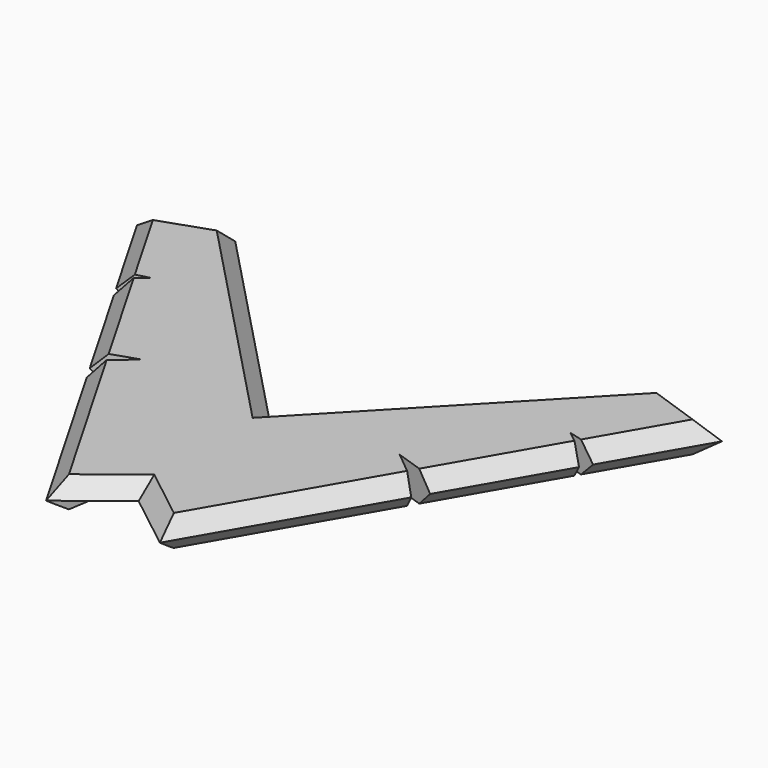
from build123d import *

# Parameters (mm, degrees)
F1_DEPTH = 6.35
F3_DEPTH = 3.175
F4_SIZE  = 3.17499


# Not quite as in the source:
# - a fillet or chamfer is up to 0.001 mm smaller than in the source, because OpenCascade refuses the exact size


with BuildPart() as f1:
    # F0 (on Top) → F1 (new body)
    with BuildSketch(Plane.XY):
        Polygon((-21.1028610796, 36.5512275749), (-11.7370359251, 20.3291425525), (0, 29.516665265), (11.7370359251, 20.3291425525), (33.4666037048, 57.9658579735), (26.5181194991, 63.6764243245), (35.1014384706, 60.7974748498), (47.9729409095, 83.0915710438), (43.2239025831, 86.8056491017), (49.1863254635, 85.1932147405), (60.325, 104.4859649666), (44.45, 109.9852262806), (0, 63.5), (-44.45, 109.9852262806), (-60.325, 104.4859649666), (-49.1863254635, 85.1932147405), (-43.2239025831, 86.8056491017), (-47.9729409095, 83.0915710438), (-35.1014384706, 60.7974748498), (-26.5181194991, 63.6764243245), (-33.4666037048, 57.9658579735), align=None)
    extrude(amount=F1_DEPTH)

    # F2 (on face) → F3 (cut)
    with BuildSketch(Plane(origin=(0, 0, 0), x_dir=(1, 0, 0), z_dir=(0, 0, -1))):
        with BuildLine():
            ThreePointArc((11.7370359251, -75.7744380392), (8.6743378245, -48.0517902958), (11.7370359251, -20.3291425525))
            Line((11.7370359251, -20.3291425525), (0, -29.516665265))
            Line((0, -29.516665265), (-11.7370359251, -20.3291425525))
            ThreePointArc((-11.7370359251, -20.3291425525), (-8.6743378245, -48.0517902958), (-11.7370359251, -75.7744380392))
            Line((-11.7370359251, -75.7744380392), (0, -63.5))
            Line((0, -63.5), (11.7370359251, -75.7744380392))
        make_face()
        Polygon((-11.7370359251, -75.7744380392), (11.7370359251, -75.7744380392), (0, -63.5), align=None)
        Polygon((0, -29.516665265), (11.7370359251, -20.3291425525), (-11.7370359251, -20.3291425525), align=None)
    extrude(amount=-F3_DEPTH, mode=Mode.SUBTRACT)

    # F4 (size 3.175 in the source; OpenCascade refuses exactly that, so slightly less here)
    f4_edges = [f1.edges().sort_by_distance(p)[0] for p in [
        (22.60182, 39.1475, 6.35),
        (22.60182, 39.1475, 0),
        (41.53719, 71.944523, 6.35),
        (41.53719, 71.944523, 0),
        (54.755663, 94.83959, 6.35),
        (54.755663, 94.83959, 0),
        (52.3875, 107.235596, 6.35),
        (52.3875, 107.235596, 0),
        (22.225, 86.742613, 6.35),
        (28.093518, 92.879832, 0),
        (5.868518, 24.922904, 6.35),
        (-5.868518, 24.922904, 6.35),
        (-22.225, 86.742613, 6.35),
        (-28.093518, 92.879832, 0),
        (-52.3875, 107.235596, 6.35),
        (-52.3875, 107.235596, 0),
        (-54.755663, 94.83959, 6.35),
        (-54.755663, 94.83959, 0),
        (-41.53719, 71.944523, 6.35),
        (-41.53719, 71.944523, 0),
        (-22.60182, 39.1475, 6.35),
        (-22.60182, 39.1475, 0),
    ]]
    chamfer(f4_edges, length=F4_SIZE)


solid = f1.part
